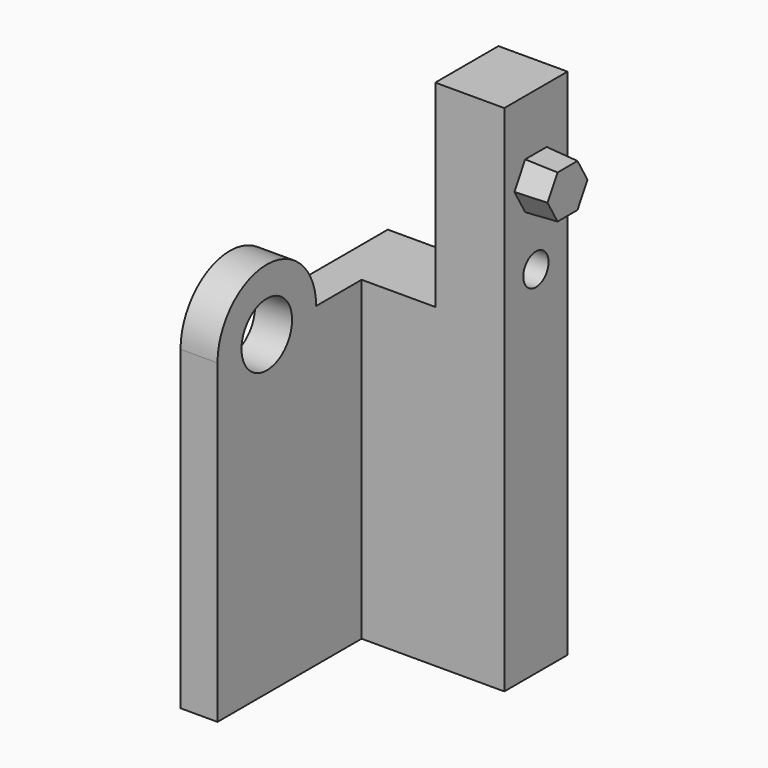
from build123d import *

# Parameters (mm, degrees)
F0_W      = 12.7
F0_H      = 50.8
F1_DEPTH  = 11.0998
F3_DEPTH  = 5.08
F3_TAPER  = 3
F4_R      = 2.54
F5_DEPTH  = 16.1808001
F6_W      = 12.7
F6_H      = 19.05
F7_DEPTH  = 17.78
F8_W      = 5.9436
F8_H      = 19.05
F9_DEPTH  = 25.4
F10_W     = 5.9436
F10_H     = 12.7
F11_DEPTH = 6.35
F12_R     = 6.34999
F13_R     = 5.08
F14_DEPTH = 33.9608001
F16_DEPTH = 5.9436
F18_DEPTH = 31.75


# Not quite as in the source:
# - a fillet or chamfer is up to 0.001 mm smaller than in the source, because OpenCascade refuses the exact size


with BuildPart() as f1:
    # F0 (on Right) → F1 (new body)
    with BuildSketch(Plane.YZ):
        with Locations((6.35, 25.4)):
            Rectangle(F0_W, F0_H)
    extrude(amount=F1_DEPTH)

    # F2 (on face) → F3 (join)
    with BuildSketch(Plane.YZ.offset(11.0998)):
        Polygon((4.191, 34.3605023065), (8.509, 34.3605023065), (10.668, 38.1), (8.509, 41.8394976935), (4.191, 41.8394976935), (2.032, 38.1), align=None)
    extrude(amount=F3_DEPTH, taper=F3_TAPER)

    # F4 (on face) → F5 (cut, through all)
    with BuildSketch(Plane(origin=(0, 0, 0), x_dir=(0, -1, 0), z_dir=(-1, 0, 0))):
        with Locations((-6.35, 25.4)):
            Circle(F4_R)
    extrude(amount=-F5_DEPTH, mode=Mode.SUBTRACT)

    # F6 (on face) → F7 (join)
    with BuildSketch(Plane(origin=(0, 0, 0), x_dir=(0, -1, 0), z_dir=(-1, 0, 0))):
        with Locations((-6.35, 9.525)):
            Rectangle(F6_W, F6_H)
    extrude(amount=F7_DEPTH)

    # F8 (on face) → F9 (join)
    with BuildSketch(Plane.XZ):
        with Locations((-14.8082, 9.525)):
            Rectangle(F8_W, F8_H)
    extrude(amount=F9_DEPTH)

    # F10 (on face) → F11 (join)
    with BuildSketch(Plane.XY.offset(19.05)):
        with Locations((-14.8082, -19.05)):
            Rectangle(F10_W, F10_H)
    extrude(amount=F11_DEPTH)

    # F12 (radius 6.35 in the source; OpenCascade refuses exactly that, so slightly less here)
    f12_edges = [f1.edges().sort_by_distance(p)[0] for p in [
        (-14.8082, -12.7, 25.4),
        (-14.8082, -25.4, 25.4),
    ]]
    fillet(f12_edges, radius=F12_R)

    # F13 (on face) → F14 (cut, through all)
    with BuildSketch(Plane(origin=(-17.78, 0, 0), x_dir=(0, -1, 0), z_dir=(-1, 0, 0))):
        with Locations((19.05, 19.05)):
            Circle(F13_R)
    extrude(amount=-F14_DEPTH, mode=Mode.SUBTRACT)

    # F15 (on face) → F16 (join, through all)
    with BuildSketch(Plane(origin=(-17.78, 0, 0), x_dir=(0, -1, 0), z_dir=(-1, 0, 0))):
        with BuildLine():
            Line((28.956, 0), (28.956, 19.05))
            ThreePointArc((28.956, 19.05), (19.05, 28.956), (9.144, 19.05))
            Line((9.144, 19.05), (12.7, 19.05))
            ThreePointArc((12.7, 19.05), (19.05, 25.4), (25.4, 19.05))
            Line((25.4, 19.05), (25.4, 0))
            Line((25.4, 0), (28.956, 0))
        make_face()
    extrude(amount=-F16_DEPTH)

    # F17 (on face) → F18 (join)
    with BuildSketch(Plane(origin=(0, 0, 0), x_dir=(1, 0, 0), z_dir=(0, 0, -1))):
        Polygon((-17.78, -12.7), (11.0998, -12.7), (11.0998, 0), (-11.8364, 0), (-11.8364, 28.956), (-17.78, 28.956), align=None)
    extrude(amount=F18_DEPTH)


solid = f1.part
